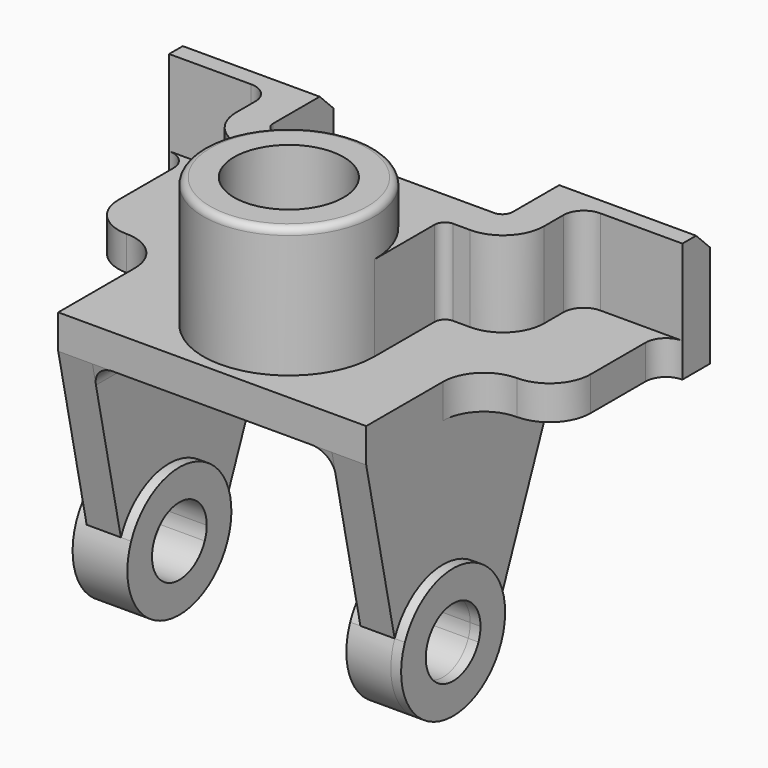
from build123d import *

# Parameters (mm, degrees)
F0_R          = 16
F1_DEPTH      = 10
F2_DEPTH      = 35
F3_DEPTH      = 48
F5_DEPTH      = 10
F6_DEPTH      = 3
F6_DEPTH_BACK = 13
F7_T4_DEPTH   = 103
F7_S5_R       = 25
F7_T6_DEPTH   = 53
F7_T11_DEPTH  = 103
F7_S12_R      = 25
F7_T13_DEPTH  = 53
F13_R         = 2
F14_SIZE      = 5


# Not quite as in the source:
# - a fillet or chamfer that OpenCascade refuses, or shapes differently, is made with other operations: its cross-section is extruded or revolved along the edge and cut away or added
# - a feature of the source that left no trace in its solid (it failed there, or was rolled back) is left out
# - a pattern or mirror of a feature is missing from the dataset's text; its kind, count and spacing are read off the source's solid


with BuildPart() as f1:
    # F0 (on Top) → F1 (new body)
    with BuildSketch(Plane.XY):
        with BuildLine():
            Line((-42.0465118704, 47.3822976644), (-82.0465118704, 47.3822976644))
            Line((-82.0465118704, 47.3822976644), (-82.0465118704, 37.3822976644))
            Line((-82.0465118704, 37.3822976644), (-58.0465118704, 37.3822976644))
            ThreePointArc((-58.0465118704, 37.3822976644), (-53.8038711833, 35.6249383515), (-52.0465118704, 31.3822976644))
            Line((-52.0465118704, 31.3822976644), (-52.0465118704, 24.3822976644))
            ThreePointArc((-52.0465118704, 24.3822976644), (-48.5317932447, 15.8970162901), (-40.0465118704, 12.3822976644))
            Line((-40.0465118704, 12.3822976644), (-35.0465118704, 12.3822976644))
            ThreePointArc((-35.0465118704, 12.3822976644), (-32.9251915269, 11.5036180079), (-32.0465118704, 9.3822976644))
            Line((-32.0465118704, 9.3822976644), (-32.0465118704, -12.6177023356))
            ThreePointArc((-32.0465118704, -12.6177023356), (-7.0465118704, 12.3822976644), (17.9534881296, -12.6177023356))
            Line((17.9534881296, -12.6177023356), (17.9534881296, 9.3822976644))
            ThreePointArc((17.9534881296, 9.3822976644), (18.832167786, 11.5036180079), (20.9534881296, 12.3822976644))
            Line((20.9534881296, 12.3822976644), (25.9534881296, 12.3822976644))
            ThreePointArc((25.9534881296, 12.3822976644), (34.4387695038, 15.8970162901), (37.9534881296, 24.3822976644))
            Line((37.9534881296, 24.3822976644), (37.9534881296, 31.3822976644))
            ThreePointArc((37.9534881296, 31.3822976644), (39.7108474424, 35.6249383515), (43.9534881296, 37.3822976644))
            Line((43.9534881296, 37.3822976644), (67.9534881296, 37.3822976644))
            Line((67.9534881296, 37.3822976644), (67.9534881296, 47.3822976644))
            Line((67.9534881296, 47.3822976644), (27.9534881296, 47.3822976644))
            Line((27.9534881296, 47.3822976644), (27.9534881296, 25.3822976644))
            ThreePointArc((27.9534881296, 25.3822976644), (27.0748084731, 23.2609773208), (24.9534881296, 22.3822976644))
            Line((24.9534881296, 22.3822976644), (-39.0465118704, 22.3822976644))
            ThreePointArc((-39.0465118704, 22.3822976644), (-41.167832214, 23.2609773208), (-42.0465118704, 25.3822976644))
            Line((-42.0465118704, 25.3822976644), (-42.0465118704, 47.3822976644))
        make_face()
        with BuildLine():
            Line((27.9534881296, 47.3822976644), (-42.0465118704, 47.3822976644))
            Line((-42.0465118704, 47.3822976644), (-42.0465118704, 25.3822976644))
            ThreePointArc((-42.0465118704, 25.3822976644), (-41.167832214, 23.2609773208), (-39.0465118704, 22.3822976644))
            Line((-39.0465118704, 22.3822976644), (24.9534881296, 22.3822976644))
            ThreePointArc((24.9534881296, 22.3822976644), (27.0748084731, 23.2609773208), (27.9534881296, 25.3822976644))
            Line((27.9534881296, 25.3822976644), (27.9534881296, 47.3822976644))
        make_face()
        with BuildLine():
            Line((-58.0465118704, 37.3822976644), (-82.0465118704, 37.3822976644))
            ThreePointArc((-82.0465118704, 37.3822976644), (-77.8038711833, 35.6249383515), (-76.0465118704, 31.3822976644))
            Line((-76.0465118704, 31.3822976644), (-76.0465118704, 11.3822976644))
            ThreePointArc((-76.0465118704, 11.3822976644), (-72.5317932447, 2.8970162901), (-64.0465118704, -0.6177023356))
            ThreePointArc((-64.0465118704, -0.6177023356), (-55.5612304962, -4.1324209614), (-52.0465118704, -12.6177023356))
            Line((-52.0465118704, -12.6177023356), (-52.0465118704, -40.6177023356))
            Line((-52.0465118704, -40.6177023356), (37.9534881296, -40.6177023356))
            Line((37.9534881296, -40.6177023356), (37.9534881296, -12.6177023356))
            ThreePointArc((37.9534881296, -12.6177023356), (41.4682067553, -4.1324209614), (49.9534881296, -0.6177023356))
            ThreePointArc((49.9534881296, -0.6177023356), (58.4387695038, 2.8970162901), (61.9534881296, 11.3822976644))
            Line((61.9534881296, 11.3822976644), (61.9534881296, 31.3822976644))
            ThreePointArc((61.9534881296, 31.3822976644), (63.7108474424, 35.6249383515), (67.9534881296, 37.3822976644))
            Line((67.9534881296, 37.3822976644), (43.9534881296, 37.3822976644))
            ThreePointArc((43.9534881296, 37.3822976644), (39.7108474424, 35.6249383515), (37.9534881296, 31.3822976644))
            Line((37.9534881296, 31.3822976644), (37.9534881296, 24.3822976644))
            ThreePointArc((37.9534881296, 24.3822976644), (34.4387695038, 15.8970162901), (25.9534881296, 12.3822976644))
            Line((25.9534881296, 12.3822976644), (20.9534881296, 12.3822976644))
            ThreePointArc((20.9534881296, 12.3822976644), (18.832167786, 11.5036180079), (17.9534881296, 9.3822976644))
            Line((17.9534881296, 9.3822976644), (17.9534881296, -12.6177023356))
            ThreePointArc((17.9534881296, -12.6177023356), (-7.0465118704, -37.6177023356), (-32.0465118704, -12.6177023356))
            Line((-32.0465118704, -12.6177023356), (-32.0465118704, 9.3822976644))
            ThreePointArc((-32.0465118704, 9.3822976644), (-32.9251915269, 11.5036180079), (-35.0465118704, 12.3822976644))
            Line((-35.0465118704, 12.3822976644), (-40.0465118704, 12.3822976644))
            ThreePointArc((-40.0465118704, 12.3822976644), (-48.5317932447, 15.8970162901), (-52.0465118704, 24.3822976644))
            Line((-52.0465118704, 24.3822976644), (-52.0465118704, 31.3822976644))
            ThreePointArc((-52.0465118704, 31.3822976644), (-53.8038711833, 35.6249383515), (-58.0465118704, 37.3822976644))
        make_face()
        with BuildLine():
            ThreePointArc((17.9534881296, -12.6177023356), (-7.0465118704, 12.3822976644), (-32.0465118704, -12.6177023356))
            ThreePointArc((-32.0465118704, -12.6177023356), (-7.0465118704, -37.6177023356), (17.9534881296, -12.6177023356))
        make_face()
        with Locations((-7.0465118704, -12.6177023356)):
            Circle(F0_R, mode=Mode.SUBTRACT)
    extrude(amount=F1_DEPTH)

    # F0 (on Top) → F2 (join)
    with BuildSketch(Plane.XY):
        with BuildLine():
            Line((-42.0465118704, 47.3822976644), (-82.0465118704, 47.3822976644))
            Line((-82.0465118704, 47.3822976644), (-82.0465118704, 37.3822976644))
            Line((-82.0465118704, 37.3822976644), (-58.0465118704, 37.3822976644))
            ThreePointArc((-58.0465118704, 37.3822976644), (-53.8038711833, 35.6249383515), (-52.0465118704, 31.3822976644))
            Line((-52.0465118704, 31.3822976644), (-52.0465118704, 24.3822976644))
            ThreePointArc((-52.0465118704, 24.3822976644), (-48.5317932447, 15.8970162901), (-40.0465118704, 12.3822976644))
            Line((-40.0465118704, 12.3822976644), (-35.0465118704, 12.3822976644))
            ThreePointArc((-35.0465118704, 12.3822976644), (-32.9251915269, 11.5036180079), (-32.0465118704, 9.3822976644))
            Line((-32.0465118704, 9.3822976644), (-32.0465118704, -12.6177023356))
            ThreePointArc((-32.0465118704, -12.6177023356), (-7.0465118704, 12.3822976644), (17.9534881296, -12.6177023356))
            Line((17.9534881296, -12.6177023356), (17.9534881296, 9.3822976644))
            ThreePointArc((17.9534881296, 9.3822976644), (18.832167786, 11.5036180079), (20.9534881296, 12.3822976644))
            Line((20.9534881296, 12.3822976644), (25.9534881296, 12.3822976644))
            ThreePointArc((25.9534881296, 12.3822976644), (34.4387695038, 15.8970162901), (37.9534881296, 24.3822976644))
            Line((37.9534881296, 24.3822976644), (37.9534881296, 31.3822976644))
            ThreePointArc((37.9534881296, 31.3822976644), (39.7108474424, 35.6249383515), (43.9534881296, 37.3822976644))
            Line((43.9534881296, 37.3822976644), (67.9534881296, 37.3822976644))
            Line((67.9534881296, 37.3822976644), (67.9534881296, 47.3822976644))
            Line((67.9534881296, 47.3822976644), (27.9534881296, 47.3822976644))
            Line((27.9534881296, 47.3822976644), (27.9534881296, 25.3822976644))
            ThreePointArc((27.9534881296, 25.3822976644), (27.0748084731, 23.2609773208), (24.9534881296, 22.3822976644))
            Line((24.9534881296, 22.3822976644), (-39.0465118704, 22.3822976644))
            ThreePointArc((-39.0465118704, 22.3822976644), (-41.167832214, 23.2609773208), (-42.0465118704, 25.3822976644))
            Line((-42.0465118704, 25.3822976644), (-42.0465118704, 47.3822976644))
        make_face()
        with BuildLine():
            ThreePointArc((17.9534881296, -12.6177023356), (-7.0465118704, 12.3822976644), (-32.0465118704, -12.6177023356))
            ThreePointArc((-32.0465118704, -12.6177023356), (-7.0465118704, -37.6177023356), (17.9534881296, -12.6177023356))
        make_face()
        with Locations((-7.0465118704, -12.6177023356)):
            Circle(F0_R, mode=Mode.SUBTRACT)
    extrude(amount=F2_DEPTH)

    # F0 (on Top) → F3 (join)
    with BuildSketch(Plane.XY):
        with BuildLine():
            ThreePointArc((17.9534881296, -12.6177023356), (-7.0465118704, 12.3822976644), (-32.0465118704, -12.6177023356))
            ThreePointArc((-32.0465118704, -12.6177023356), (-7.0465118704, -37.6177023356), (17.9534881296, -12.6177023356))
        make_face()
        with Locations((-7.0465118704, -12.6177023356)):
            Circle(F0_R, mode=Mode.SUBTRACT)
    extrude(amount=F3_DEPTH)

    # F4 (on face) → F5 (join)
    with BuildSketch(Plane.YZ.offset(37.9534881296)):
        with BuildLine():
            Line((-40.6177023356, 0), (-30.2316619949, -48.8762071112))
            ThreePointArc((-30.2316619949, -48.8762071112), (-8.9890134213, -37.3497287751), (6.3822976644, -56))
            ThreePointArc((6.3822976644, -56), (6.0325688893, -59.6286889144), (4.9962573236, -63.1237928888))
            Line((4.9962573236, -63.1237928888), (24.2060349548, -15.6265883042))
            ThreePointArc((24.2060349548, -15.6265883042), (33.4061625118, -4.2715739575), (47.3822976644, 0))
            Line((47.3822976644, 0), (36.7724023624, 0))
            Line((36.7724023624, 0), (-12.6177023356, 0))
            Line((-12.6177023356, 0), (-40.6177023356, 0))
        make_face()
    f5 = extrude(amount=-F5_DEPTH)

    # F5_copies: F5 across plane
    add(f5.mirror(Plane(origin=(-7.046512, 0, 0), x_dir=(0, 0, -1), z_dir=(-1, 0, 0))))

    # F4 (on face) → F6 (join, two sides)
    with BuildSketch(Plane.YZ.offset(37.9534881296)) as f6_sk:
        with BuildLine():
            ThreePointArc((-3.3471972518, -59.7493646783), (-16.367067014, -65.2705050838), (-21.8882074194, -52.2506353217))
            Line((-21.8882074194, -52.2506353217), (-30.2316619949, -48.8762071112))
            ThreePointArc((-30.2316619949, -48.8762071112), (-19.7414952245, -73.6139596592), (4.9962573236, -63.1237928888))
            Line((4.9962573236, -63.1237928888), (-3.3471972518, -59.7493646783))
        make_face()
        with BuildLine():
            ThreePointArc((-21.8882074194, -52.2506353217), (-10.7078660649, -46.1840677764), (-2.6177023356, -56))
            ThreePointArc((-2.6177023356, -56), (-2.801770112, -57.9098362707), (-3.3471972518, -59.7493646783))
            Line((-3.3471972518, -59.7493646783), (4.9962573236, -63.1237928888))
            ThreePointArc((4.9962573236, -63.1237928888), (6.0325688893, -59.6286889144), (6.3822976644, -56))
            ThreePointArc((6.3822976644, -56), (-8.9890134213, -37.3497287751), (-30.2316619949, -48.8762071112))
            Line((-30.2316619949, -48.8762071112), (-21.8882074194, -52.2506353217))
        make_face()
    f6 = extrude(amount=F6_DEPTH) + extrude(f6_sk.sketch, amount=-F6_DEPTH_BACK)

    # F6_copies: F6 across plane
    add(f6.mirror(Plane(origin=(-7.046512, 0, 0), x_dir=(0, 0, -1), z_dir=(-1, 0, 0))))

    # F7: fillet of radius 6 on 2 edges, made by hand


with BuildPart() as f7_tool2:
    # F7_s3 → F7_t4 (new body)
    with BuildSketch(Plane.XZ.offset(-47.3822976644)):
        with BuildLine():
            ThreePointArc((21.9534881296, 0), (26.1961288167, -1.7573593129), (27.9534881296, -6))
            Line((27.9534881296, -6), (27.9534881296, 0))
            Line((27.9534881296, 0), (21.9534881296, 0))
        make_face()
    extrude(amount=F7_T4_DEPTH)

    # F7_s5 → F7_t6 (cut, symmetric)
    with BuildSketch(Plane.YZ.offset(25)):
        with Locations((47.3822976644, -25)):
            Circle(F7_S5_R)
    extrude(amount=F7_T6_DEPTH, both=True, mode=Mode.SUBTRACT)

    split(bisect_by=Plane(origin=(0, -38.8628535351, -8.2582341886), x_dir=(1, 0, 0), z_dir=(0, 0.9781594762, 0.2078558133)), keep=Keep.TOP)


with BuildPart() as f1_1:
    add(f1.part)

    # F7_t1: union F7_tool2
    add(f7_tool2.part)


with BuildPart() as f7_tool9:
    # F7_s10 → F7_t11 (new body)
    with BuildSketch(Plane.XZ.offset(-47.3822976644)):
        with BuildLine():
            ThreePointArc((-36.0465121296, 0), (-40.2891528167, -1.7573593129), (-42.0465121296, -6))
            Line((-42.0465121296, -6), (-42.0465121296, 0))
            Line((-42.0465121296, 0), (-36.0465121296, 0))
        make_face()
    extrude(amount=F7_T11_DEPTH)

    # F7_s12 → F7_t13 (cut, symmetric)
    with BuildSketch(Plane.YZ.offset(-39)):
        with Locations((47.3822976644, -25)):
            Circle(F7_S12_R)
    extrude(amount=F7_T13_DEPTH, both=True, mode=Mode.SUBTRACT)

    split(bisect_by=Plane(origin=(0, -38.8628535351, -8.2582341886), x_dir=(1, 0, 0), z_dir=(0, 0.9781594762, 0.2078558133)), keep=Keep.TOP)


with BuildPart() as f1_2:
    add(f1_1.part)

    # F7_t8: union F7_tool9
    add(f7_tool9.part)

    # F13
    f13_edges = [f1_2.edges().sort_by_distance(p)[0] for p in [
        (-32.046512, -12.617702, 48),
    ]]
    fillet(f13_edges, radius=F13_R)

    # F14
    f14_edges = [f1_2.edges().sort_by_distance(p)[0] for p in [
        (47.953488, 47.382298, 35),
        (-62.046512, 47.382298, 35),
    ]]
    chamfer(f14_edges, length=F14_SIZE)


solid = f1_2.part
